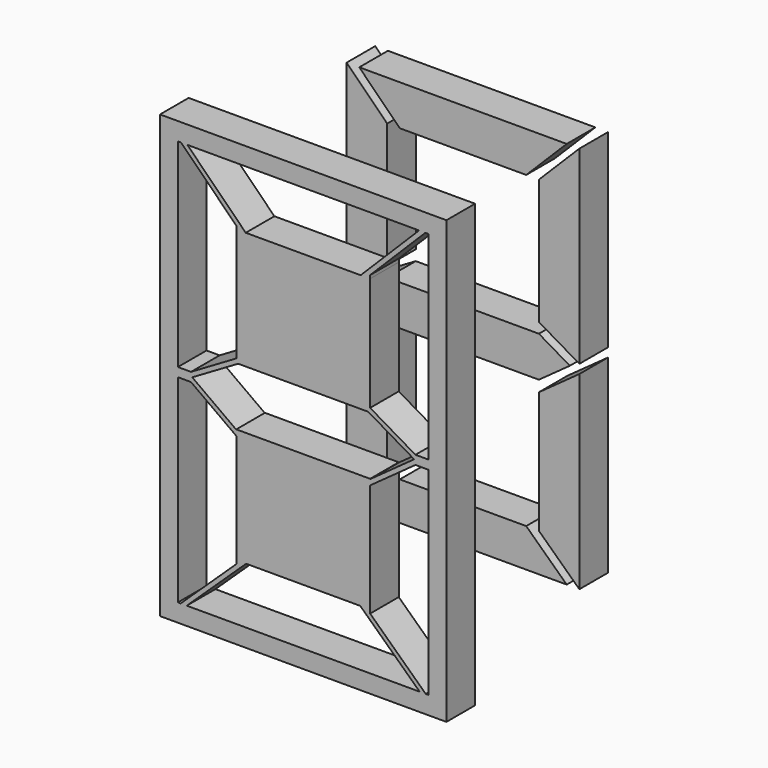
from build123d import *

# Parameters (mm, degrees)
F1_DEPTH = 25.4
F3_W     = 203.2396654825
F3_H     = 313.3949062689
F4_DEPTH = 25.4


# Not quite as in the source:
# - a feature names something its author has since deleted; it is built from what else it names


with BuildPart() as f1:
    # F0 (on Front) → F1 (new body)
    with BuildSketch(Plane.XZ):
        Polygon((-15.1739238592, -61.2904866815), (13.5534761408, -44.45), (13.5534761408, 44.45), (-15.1739238592, 73.1868195874), align=None)
    extrude(amount=F1_DEPTH)


with BuildPart() as f1b:
    # F0 (on Front) → F1, piece 2 (new body)
    with BuildSketch(Plane.XZ):
        Polygon((140.9854855022, 73.1868195874), (-6.195139428, 73.1868195874), (22.532260572, 44.45), (112.2486659148, 44.45), align=None)
    extrude(amount=F1_DEPTH)


with BuildPart() as f1c:
    # F0 (on Front) → F1, piece 3 (new body)
    with BuildSketch(Plane.XZ):
        Polygon((149.9657416234, -61.2904866815), (149.9657416233, 73.1868195874), (121.2289220359, 44.45), (121.228922036, -44.45), align=None)
    extrude(amount=F1_DEPTH)


with BuildPart() as f1d:
    # F0 (on Front) → F1, piece 4 (new body)
    with BuildSketch(Plane.XZ):
        Polygon((121.228922036, -174.8955888238), (149.9657416234, -202.1080866815), (149.9657416234, -67.6404866815), (121.228922036, -88.3673402517), align=None)
    extrude(amount=F1_DEPTH)


with BuildPart() as f1e:
    # F0 (on Front) → F1, piece 5 (new body)
    with BuildSketch(Plane.XZ):
        Polygon((13.5534761408, -88.368464908), (-15.1739238592, -67.6404866815), (-15.1739238592, -202.1080866815), (13.5534761408, -174.8955888238), align=None)
    extrude(amount=F1_DEPTH)


with BuildPart() as f1f:
    # F0 (on Front) → F1, piece 6 (new body)
    with BuildSketch(Plane.XZ):
        Polygon((22.532260572, -174.8955888238), (-6.195139428, -202.1080866815), (140.9854855022, -202.1080866815), (112.2486659148, -174.8955888238), align=None)
    extrude(amount=F1_DEPTH)


with BuildPart() as f1g:
    # F0 (on Front) → F1, piece 7 (new body)
    with BuildSketch(Plane.XZ):
        Polygon((13.5534761408, -51.8106613985), (-8.4134451263, -64.6880413574), (13.5534761408, -80.5380613985), (121.2287825639, -80.5380613985), (143.2040990216, -64.6880413574), (121.2299748981, -51.8106613985), align=None)
    extrude(amount=F1_DEPTH)


with BuildPart() as f4:
    # F3 (on offset) → F4 (new body)
    with BuildSketch(Plane.XZ.offset(141.732)):
        with Locations((67.3959088821, -64.460633547)):
            Rectangle(F3_W, F3_H)
        Polygon((-21.5239238592, 79.5368195874), (-19.2591887281, 79.5368195874), (-14.8057116502, 79.5368195874), (149.5985100447, 79.5368195874), (154.0527170808, 79.5368195874), (156.3157416234, 79.5368195874), (156.3157416234, -61.4293413488), (156.3157416234, -67.7793413488), (156.3157416234, -208.4580866815), (154.3441700366, -208.4580866815), (150.0184539651, -208.4580866815), (-15.22550768, -208.4580866815), (-19.550556387, -208.4580866815), (-21.5239238592, -208.4580866815), (-21.5239238592, -67.7793892541), (-21.5239238592, -61.4293413488), align=None, mode=Mode.SUBTRACT)
        Polygon((19.9034761408, 40.3613134539), (19.9034761408, 38.1), (19.9034761408, -42.5824095103), (-12.2466249778, -61.4293413488), (-21.5239238592, -61.4293413488), (-21.5239238592, -67.7793892541), (-12.2466249778, -67.7793892541), (19.9034761408, -90.9769844408), (19.9034761408, -168.5455888238), (19.9034761408, -171.0846113359), (-19.550556387, -208.4580866815), (-15.22550768, -208.4580866815), (26.9088930999, -168.5455888237), (107.8702375016, -168.5455888238), (150.0184539651, -208.4580866815), (154.3441700366, -208.4580866815), (114.878922036, -171.0862413594), (114.878922036, -168.5455888238), (114.878922036, -90.974367478), (147.0377482149, -67.7793413488), (156.3157416234, -67.7793413488), (156.3157416234, -61.4293413488), (147.0377482149, -61.4293413488), (114.878922036, -42.5834742092), (114.878922036, 38.1), (114.8789220359, 40.3630245425), (154.0527170808, 79.5368195874), (149.5985100447, 79.5368195874), (108.1616904574, 38.1), (26.617525441, 38.1), (-14.8057116502, 79.5368195874), (-19.2591887281, 79.5368195874), align=None)
        Polygon((-11.340707376, -64.549165216), (21.2214801035, -45.4606613985), (113.5591913096, -45.4606613985), (146.13209243, -64.5491866901), (114.878922036, -87.090995271), (114.878922036, -86.8880613985), (19.9034761408, -86.8880613985), (19.9034761408, -87.0931043), align=None, mode=Mode.SUBTRACT)
    extrude(amount=F4_DEPTH)


solid = Compound([f1.part, f1b.part, f1c.part, f1d.part, f1e.part, f1f.part, f1g.part, f4.part])
